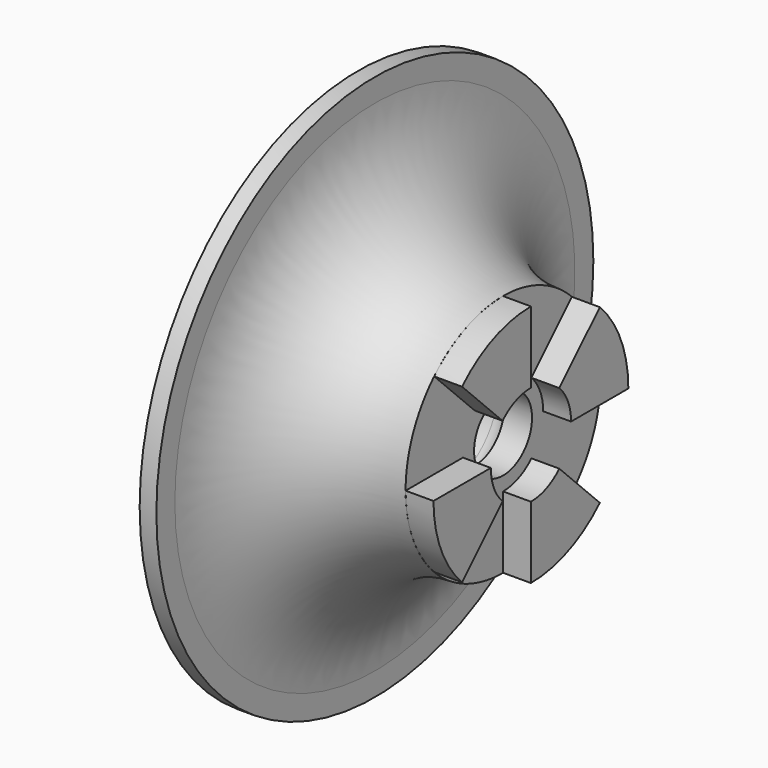
from build123d import *

# Parameters (mm, degrees)
F3_R     = 78.8340785065
F4_DEPTH = 40
F6_DEPTH = 5
F7_R     = 4.99999


# Not quite as in the source:
# - a fillet or chamfer that OpenCascade refuses, or shapes differently, is made with other operations: its cross-section is extruded or revolved along the edge and cut away or added
# - a fillet or chamfer is up to 0.001 mm smaller than in the source, because OpenCascade refuses the exact size
# - ends of sketch curves that miss each other by under 0.0002 mm in the source are joined
# - a feature names something its author has since deleted; it is built from what else it names


with BuildPart() as f1:
    # F0 (on Top) → F1 (revolve)
    with BuildSketch(Plane.XY):
        with BuildLine():
            Line((0, -49), (0, -9))
            Line((0, -9), (-31, -9))
            Line((-31, -9), (-31, -6.5))
            Line((-31, -6.5), (-36, -6.5))
            Line((-36, -6.5), (-36, -11.5))
            Line((-36, -11.5), (-57.0000335574, -11.5))
            Line((-57.0000335574, -11.5), (-57.0000000106, -49))
            Line((-57.0000000106, -49), (-54.0000000106, -49))
            Line((-54.0000000106, -49), (-54.0000000106, -44.8544277911))
            ThreePointArc((-54.0000000106, -44.8544277911), (-47.2635467929, -28.5904424478), (-31, -21.8529305247))
            Line((-31, -21.8529305247), (-26.0000000106, -21.8529305247))
            ThreePointArc((-26.0000000106, -21.8529305247), (-9.7364532177, -28.5904424478), (-3, -44.8544277911))
            Line((-3, -44.8544277911), (-3, -49))
            Line((-3, -49), (0, -49))
        make_face()
    revolve(axis=Axis((7.519562263, 0, 0), (1, 0, 0)))

    # F2: fillet of radius 5 on 1 edges, made by hand

    # F2_s1 → F2_t2 (revolve, cut)
    with BuildSketch(Plane.XY):
        with BuildLine():
            ThreePointArc((-3.0028205283, -44.4942267471), (-2.1641233212, -47.188770834), (0, -49))
            Line((0, -49), (-0.1996566353, -49.458407273))
            ThreePointArc((-0.1996566353, -49.458407273), (-1.5, -49.5), (-3, -49.5))
            Line((-3, -49.5), (-3.5, -49))
            ThreePointArc((-3.5, -49), (-3.5, -44.8544277911), (-3.5027592164, -44.5020566949))
            Line((-3.5027592164, -44.5020566949), (-3.0028205283, -44.4942267471))
        make_face()
    revolve(axis=Axis((-3, 0, 0), (1, 0, 0)), mode=Mode.SUBTRACT)

    # F3 (on face) → F4 (cut)
    with BuildSketch(Plane.YZ.offset(-31)):
        Circle(F3_R)
    extrude(amount=F4_DEPTH, mode=Mode.SUBTRACT)

    # F5 (on face) → F6 (join)
    with BuildSketch(Plane.YZ.offset(-31)):
        with BuildLine():
            Line((9, 0), (21.85, 0))
            ThreePointArc((21.85, 0), (20.1867677854, 8.3616329972), (15.4502831689, 15.4502831689))
            Line((15.4502831689, 15.4502831689), (6.3639610307, 6.3639610307))
            ThreePointArc((6.3639610307, 6.3639610307), (8.3149157926, 3.4441508913), (9, 0))
        make_face()
        with BuildLine():
            Line((0, 9), (0, 21.85))
            ThreePointArc((0, 21.85), (-8.3616329972, 20.1867677854), (-15.4502831689, 15.4502831689))
            Line((-15.4502831689, 15.4502831689), (-6.3639610307, 6.3639610307))
            ThreePointArc((-6.3639610307, 6.3639610307), (-3.4441508913, 8.3149157926), (0, 9))
        make_face()
        with BuildLine():
            ThreePointArc((0, -21.85), (8.3616329972, -20.1867677854), (15.4502831689, -15.4502831689))
            Line((15.4502831689, -15.4502831689), (6.3639610307, -6.3639610307))
            ThreePointArc((6.3639610307, -6.3639610307), (3.4441508913, -8.3149157926), (0, -9))
            Line((0, -9), (0, -21.85))
        make_face()
        with BuildLine():
            ThreePointArc((-21.85, 0), (-20.1867677854, -8.3616329972), (-15.4502831689, -15.4502831689))
            Line((-15.4502831689, -15.4502831689), (-6.3639610307, -6.3639610307))
            ThreePointArc((-6.3639610307, -6.3639610307), (-8.3149157926, -3.4441508913), (-9, 0))
            Line((-9, 0), (-21.85, 0))
        make_face()
    extrude(amount=F6_DEPTH)

    # F7 (radius 5 in the source; OpenCascade refuses exactly that, so slightly less here)
    f7_edges = [f1.edges().sort_by_distance(p)[0] for p in [
        (-36, 11.5, 0),
    ]]
    fillet(f7_edges, radius=F7_R)


solid = f1.part
